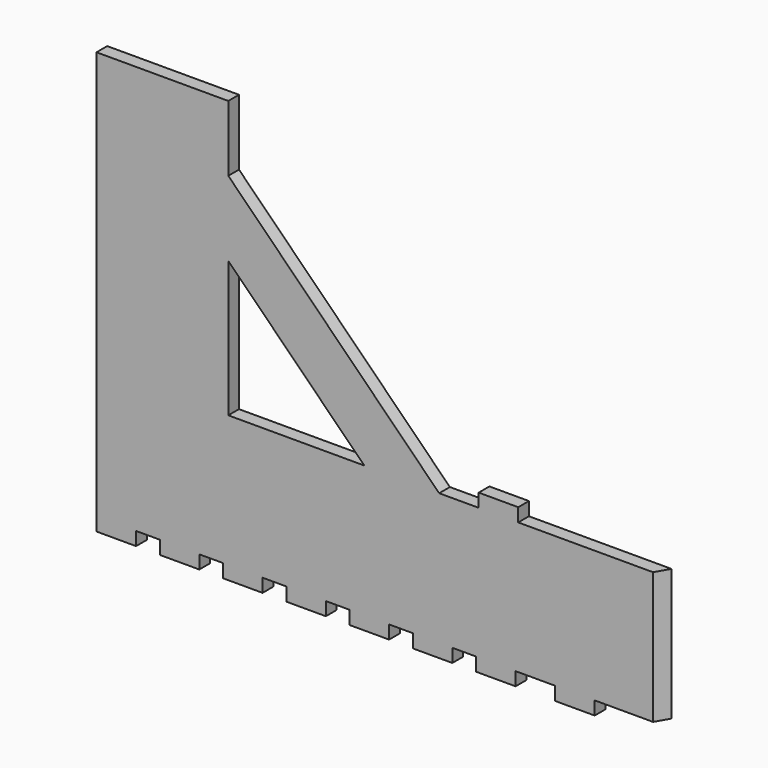
from build123d import *

# Parameters (mm, degrees)
F0_W     = 15
F0_H     = 5.08
F1_DEPTH = 5.08
F2_DEPTH = 25
F4_DEPTH = 55.7
F5_W     = 15
F5_H     = 5.08
F6_DEPTH = 5.08
F7_W     = 15
F7_H     = 5.08
F8_DEPTH = 5.08


# Not quite as in the source:
# - a feature names something its author has since deleted; it is built from what else it names


with BuildPart() as f1:
    # F0 (on Front) → F1 (new body)
    with BuildSketch(Plane.XZ):
        Polygon((-87.5, 0), (-32.419, 0), (-32.419, 50), (-116.5, 50), (-144.9023774395, 50), (-196.5, 50), (-196.5, 101.5976225605), (-196.5, 130), (-246.5, 130), (-246.5, 0), (-231.5, 0), (-222.5, 0), (-207.5, 0), (-198.5, 0), (-183.5, 0), (-174.5, 0), (-159.5, 0), (-150.5, 0), (-135.5, 0), (-126.5, 0), (-111.5, 0), (-102.5, 0), align=None)
        with Locations((-95, -2.54)):
            Rectangle(F0_W, F0_H)
        Polygon((-144.9023774395, 50), (-116.5, 50), (-196.5, 130), (-196.5, 101.5976225605), align=None)
        with Locations((-119, -2.54)):
            Rectangle(F0_W, F0_H)
        with Locations((-143, -2.54)):
            Rectangle(F0_W, F0_H)
        with Locations((-239, -2.54)):
            Rectangle(F0_W, F0_H)
        with Locations((-167, -2.54)):
            Rectangle(F0_W, F0_H)
        with Locations((-215, -2.54)):
            Rectangle(F0_W, F0_H)
        with Locations((-191, -2.54)):
            Rectangle(F0_W, F0_H)
    extrude(amount=F1_DEPTH)

    # F2 (add): a face of the model
    f2_faces = [f1.faces().sort_by_distance(p)[0] for p in [
        (-221.5, -2.54, 130),
    ]]
    extrude(f2_faces, amount=F2_DEPTH)

    # F3 (on face) → F4 (cut)
    with BuildSketch(Plane(origin=(0, 0, 0), x_dir=(1, 0, 0), z_dir=(0, 0, -1))):
        Polygon((-32.419, 5.08), (-35.3519393675, 5.08), (-32.419, 0), align=None)
    extrude(amount=-F4_DEPTH, mode=Mode.SUBTRACT)

    # F5 (on face) → F6 (join)
    with BuildSketch(Plane(origin=(0, 0, 0), x_dir=(1, 0, 0), z_dir=(0, 0, -1))):
        with Locations((-65, 2.54)):
            Rectangle(F5_W, F5_H)
    extrude(amount=F6_DEPTH)

    # F7 (on face) → F8 (join)
    with BuildSketch(Plane.XY.offset(50)):
        with Locations((-94, -2.54)):
            Rectangle(F7_W, F7_H)
    extrude(amount=F8_DEPTH)


solid = f1.part
